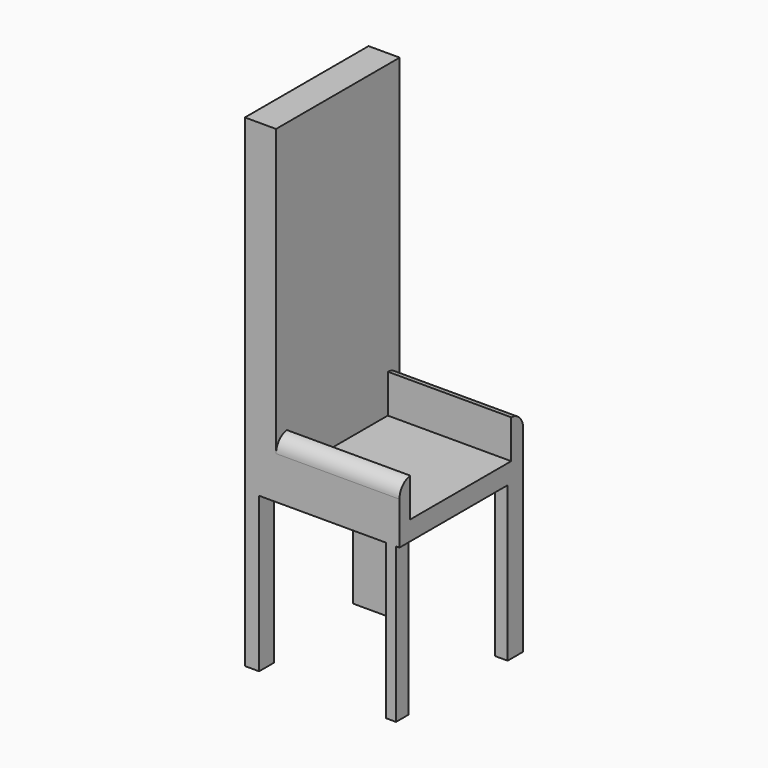
from build123d import *

# Parameters (mm, degrees)
F0_W         = 50.8
F0_H         = 50.8
F1_DEPTH     = 6.35
F2_W         = 3.2963603735
F2_H         = 5.1404060796
F2_W_2       = 4.6653077006
F2_H_2       = 6.2190000899
F2_W_3       = 4.104912895
F2_H_3       = 6.35
F2_W_4       = 12.7
F3_DEPTH     = 25.4
F4_DEPTH     = 25.4
F5_W         = 10.2360965684
F5_H         = 50.8
F6_DEPTH     = 101.6
F7_W         = 40.5639034316
F7_H         = 4.4053453021
F8_DEPTH     = 12.7
F9_W         = 40.5639034316
F9_H         = 4.8934674442
F10_DEPTH    = 12.7
F11_T1_DEPTH = 53.1514074134
F12_T1_DEPTH = 53.255338931


# Not quite as in the source:
# - a fillet or chamfer that OpenCascade refuses, or shapes differently, is made with other operations: its cross-section is extruded or revolved along the edge and cut away or added


with BuildPart() as f1:
    # F0 (on Top) → F1 (new body)
    with BuildSketch(Plane.XY):
        with Locations((25.4, 25.4)):
            Rectangle(F0_W, F0_H)
    extrude(amount=F1_DEPTH)

    # F2 (on face) → F3 (join)
    with BuildSketch(Plane(origin=(0, 0, 0), x_dir=(1, 0, 0), z_dir=(0, 0, -1))):
        with Locations((48.0348914862, -2.5702030398)):
            Rectangle(F2_W, F2_H)
        with Locations((2.3326538503, -3.109500045)):
            Rectangle(F2_W_2, F2_H_2)
        with Locations((48.7475435525, -47.625)):
            Rectangle(F2_W_3, F2_H_3)
        with Locations((6.35, -47.625)):
            Rectangle(F2_W_4, F2_H_3)
    extrude(amount=F3_DEPTH)

    # F4 (add): faces of the model
    f4_faces = [f1.faces().sort_by_distance(p)[0] for p in [
        (48.0348914862, 2.5702030398, -25.4),
        (2.3326538503, 3.109500045, -25.4),
        (6.35, 47.625, -25.4),
        (48.7475435525, 47.625, -25.4),
    ]]
    extrude(f4_faces, amount=F4_DEPTH)

    # F5 (on face) → F6 (join)
    with BuildSketch(Plane.XY.offset(6.35)):
        with Locations((5.1180482842, 25.4)):
            Rectangle(F5_W, F5_H)
    extrude(amount=F6_DEPTH)

    # F7 (on face) → F8 (join)
    with BuildSketch(Plane.XY.offset(6.35)):
        with Locations((30.5180482842, 2.202672651)):
            Rectangle(F7_W, F7_H)
    extrude(amount=F8_DEPTH)

    # F9 (on face) → F10 (join)
    with BuildSketch(Plane.XY.offset(6.35)):
        with Locations((30.5180482842, 48.3532662779)):
            Rectangle(F9_W, F9_H)
    extrude(amount=F10_DEPTH)

    # F11: fillet of radius 5.08 on 1 edges, made by hand

    # F11_s2 → F11_t1 (cut)
    with BuildSketch(Plane.YZ.offset(10.2360965684)):
        with BuildLine():
            ThreePointArc((4.4053453021, 19.05), (1.2568046175, 17.3600809275), (0, 14.0149984073))
            Line((0, 14.0149984073), (0, 19.05))
            Line((0, 19.05), (4.4053453021, 19.05))
        make_face()
    extrude(amount=F11_T1_DEPTH, mode=Mode.SUBTRACT)

    # F12: fillet of radius 5.08 on 1 edges, made by hand

    # F12_s2 → F12_t1 (cut)
    with BuildSketch(Plane.YZ.offset(10.2360965684)):
        with BuildLine():
            ThreePointArc((45.9065325558, 19.05), (49.3774571346, 17.498962257), (50.8, 13.9734258002))
            Line((50.8, 13.9734258002), (50.8, 19.05))
            Line((50.8, 19.05), (45.9065325558, 19.05))
        make_face()
    extrude(amount=F12_T1_DEPTH, mode=Mode.SUBTRACT)


solid = f1.part
